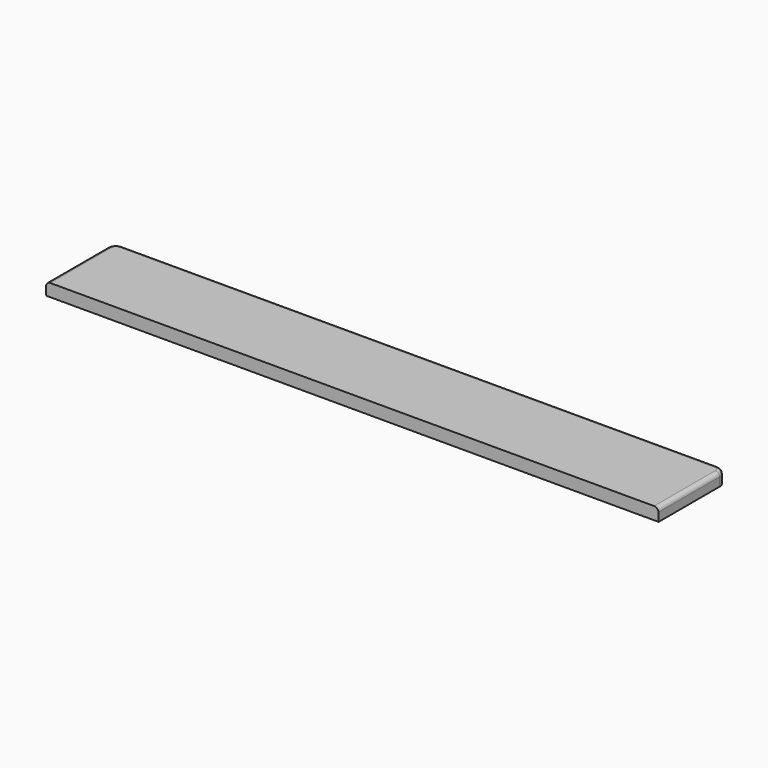
from build123d import *

# Parameters (mm, degrees)
F1_DEPTH    = 914.4
F2_R        = 6.35
F3_T1_DEPTH = 50.8
F3_T4_ANGLE = 90
F3_T6_ANGLE = 90


# Not quite as in the source:
# - a fillet or chamfer that OpenCascade refuses, or shapes differently, is made with other operations: its cross-section is extruded or revolved along the edge and cut away or added


with BuildPart() as f1:
    # F0 (on Right) → F1 (new body)
    with BuildSketch(Plane.YZ):
        Polygon((-19.769934752, -26.0955506578), (-146.769934752, -26.0955506578), (-146.2517950619, -45.1455506578), (-19.769934752, -45.1455506578), align=None)
    extrude(amount=F1_DEPTH)

    # F2
    f2_edges = [f1.edges().sort_by_distance(p)[0] for p in [
        (0, -83.269935, -26.095551),
        (457.2, -19.769935, -26.095551),
        (914.4, -83.269935, -26.095551),
    ]]
    fillet(f2_edges, radius=F2_R)

    # F3: fillet of radius 12.7 on 2 edges, made by hand

    # F3_s2 → F3_t1 (cut)
    with BuildSketch(Plane.XY.offset(-76.8955506578)):
        with BuildLine():
            ThreePointArc((914.4, -32.469934752), (910.6802561211, -23.489678631), (901.7, -19.769934752))
            Line((901.7, -19.769934752), (914.4, -19.769934752))
            Line((914.4, -19.769934752), (914.4, -32.469934752))
        make_face()
        with BuildLine():
            ThreePointArc((0, -32.469934752), (3.7197438789, -23.489678631), (12.7, -19.769934752))
            Line((12.7, -19.769934752), (0, -19.769934752))
            Line((0, -19.769934752), (0, -32.469934752))
        make_face()
    extrude(amount=F3_T1_DEPTH, mode=Mode.SUBTRACT)

    # F3_s3 → F3_t4 (revolve, cut)
    with BuildSketch(Plane.YZ.offset(12.7)):
        with BuildLine():
            ThreePointArc((-26.119934752, -26.0955506578), (-21.6298066915, -27.9554225973), (-19.769934752, -32.4455506578))
            Line((-19.769934752, -32.4455506578), (-19.769934752, -26.0955506578))
            Line((-19.769934752, -26.0955506578), (-26.119934752, -26.0955506578))
        make_face()
    revolve(axis=Axis((12.7, -32.469934752, -26.0955506578), (0, 0, 1)), revolution_arc=F3_T4_ANGLE, mode=Mode.SUBTRACT)

    # F3_s5 → F3_t6 (revolve, cut)
    with BuildSketch(Plane.XZ.offset(32.469934752)):
        with BuildLine():
            ThreePointArc((908.05, -26.0955506578), (912.5401280605, -27.9554225973), (914.4, -32.4455506578))
            Line((914.4, -32.4455506578), (914.4, -26.0955506578))
            Line((914.4, -26.0955506578), (908.05, -26.0955506578))
        make_face()
    revolve(axis=Axis((901.7, -32.469934752, -26.0955506578), (0, 0, 1)), revolution_arc=F3_T6_ANGLE, mode=Mode.SUBTRACT)


solid = f1.part
